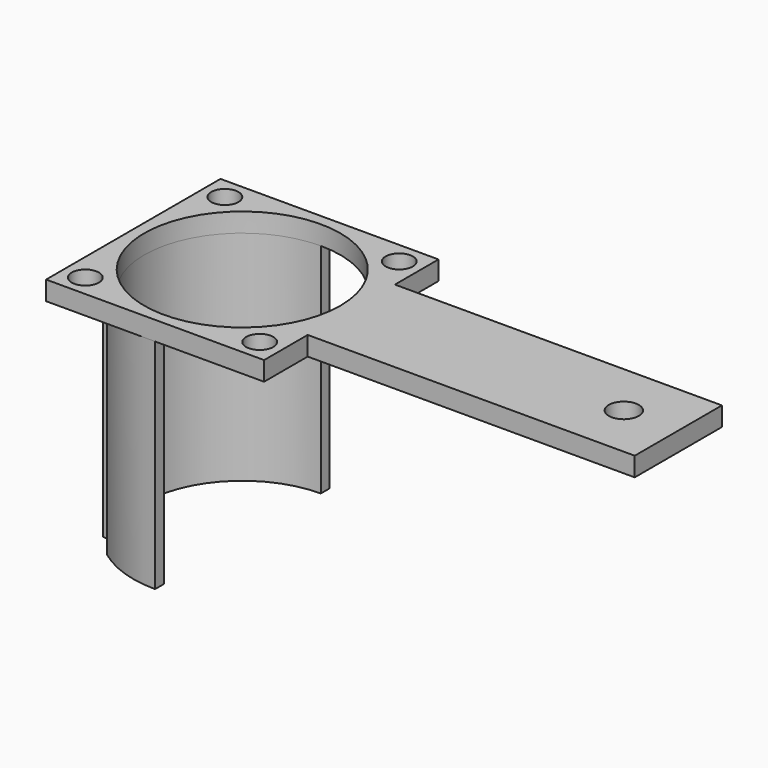
from build123d import *

# Parameters (mm, degrees)
F0_W     = 40
F0_H     = 40
F0_R     = 2.5
F0_R_2   = 18
F1_DEPTH = 3.5
F2_W     = 60
F2_H     = 20
F2_R     = 2.75
F3_DEPTH = 3.5
F7_DEPTH = 40
F8_R     = 4
F9_DEPTH = 40.001


with BuildPart() as f1:
    # F0 (on Top) → F1 (new body)
    with BuildSketch(Plane.XY):
        with Locations((20, 20)):
            Rectangle(F0_W, F0_H)
        with Locations((4, 4)):
            Circle(F0_R, mode=Mode.SUBTRACT)
        with Locations((36, 4)):
            Circle(F0_R, mode=Mode.SUBTRACT)
        with Locations((4, 36)):
            Circle(F0_R, mode=Mode.SUBTRACT)
        with Locations((20, 20)):
            Circle(F0_R_2, mode=Mode.SUBTRACT)
        with Locations((36, 36)):
            Circle(F0_R, mode=Mode.SUBTRACT)
    extrude(amount=F1_DEPTH)

    # F2 (on face) → F3 (join, through all)
    with BuildSketch(Plane.XY.offset(3.5)):
        with Locations((70, 20)):
            Rectangle(F2_W, F2_H)
        with Locations((90, 20)):
            Circle(F2_R, mode=Mode.SUBTRACT)
    extrude(amount=-F3_DEPTH)

    # F6 (on face) → F7 (join, through all)
    with BuildSketch(Plane.XY):
        with BuildLine():
            Line((20, 38), (20, 40))
            ThreePointArc((20, 40), (0, 20), (20, 0))
            Line((20, 0), (20, 2))
            ThreePointArc((20, 2), (2, 20), (20, 38))
        make_face()
    extrude(amount=-F7_DEPTH)

    # F8 (on face) → F9 (cut, through all)
    with BuildSketch(Plane.XY):
        with Locations((36, 36)):
            Circle(F8_R)
        with Locations((4, 36)):
            Circle(F8_R)
        with Locations((4, 4)):
            Circle(F8_R)
        with Locations((36, 4)):
            Circle(F8_R)
    extrude(amount=-F9_DEPTH, mode=Mode.SUBTRACT)


solid = f1.part
